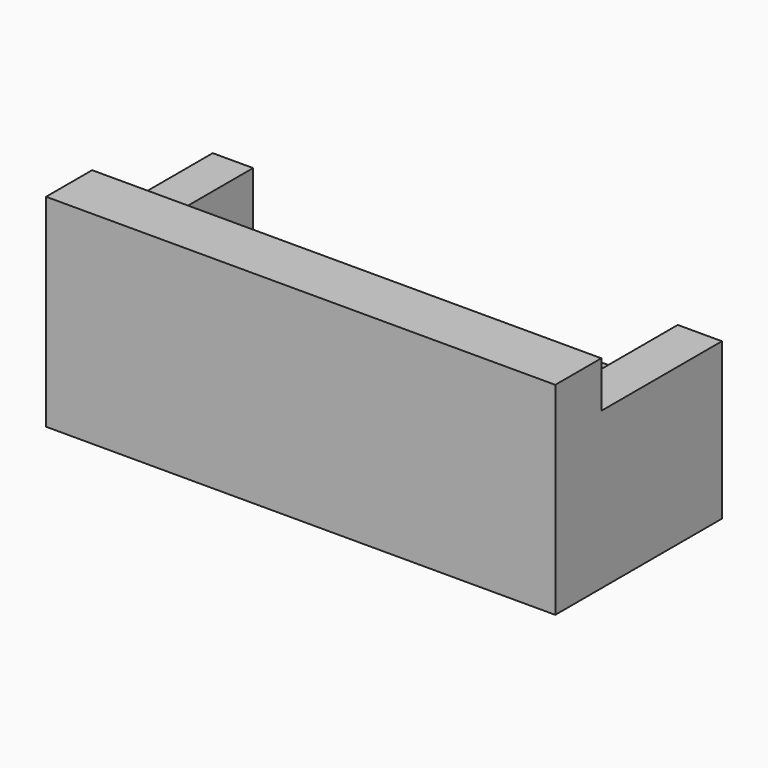
from build123d import *

# Parameters (mm, degrees)
F0_W     = 2235.2
F0_H     = 914.4
F1_DEPTH = 431.8
F2_W     = 2235.2
F2_H     = 252.5851911545
F3_DEPTH = 457.2
F4_W     = 177.183791995
F4_H     = 661.8148088455
F5_DEPTH = 254
F6_W     = 193.8291313171
F6_H     = 661.8148088455
F7_DEPTH = 254


with BuildPart() as f1:
    # F0 (on Top) → F1 (new body)
    with BuildSketch(Plane.XY):
        with Locations((1117.6, -457.2)):
            Rectangle(F0_W, F0_H)
    extrude(amount=F1_DEPTH)

    # F2 (on face) → F3 (join)
    with BuildSketch(Plane.XY.offset(431.8)):
        with Locations((1117.6, -788.1074044228)):
            Rectangle(F2_W, F2_H)
    extrude(amount=F3_DEPTH)

    # F4 (on face) → F5 (join)
    with BuildSketch(Plane.XY.offset(431.8)):
        with Locations((88.5918959975, -330.9074044228)):
            Rectangle(F4_W, F4_H)
    extrude(amount=F5_DEPTH)

    # F6 (on face) → F7 (join)
    with BuildSketch(Plane.XY.offset(431.8)):
        with Locations((2138.2854343414, -330.9074044228)):
            Rectangle(F6_W, F6_H)
    extrude(amount=F7_DEPTH)


solid = f1.part
